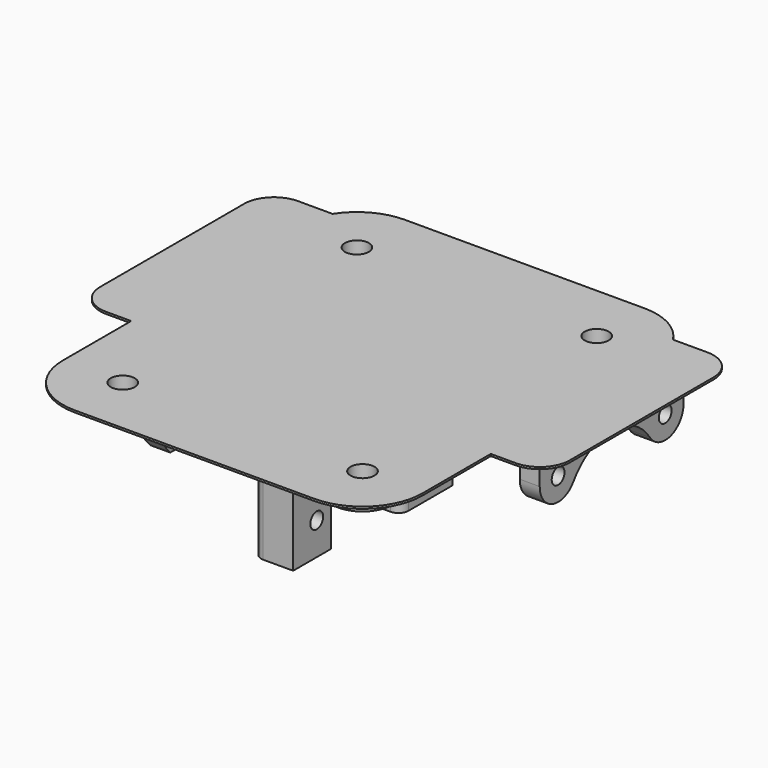
from build123d import *

# Parameters (mm, degrees)
F1_R          = 1.2
F2_DEPTH      = 2
F3_R          = 2
F4_W          = 4
F4_H          = 4.75
F5_DEPTH      = 9
F6_W          = 8.8
F6_H          = 2
F6_W_2        = 2
F6_H_2        = 6.5
F7_DEPTH      = 4
F8_R          = 0.8
F9_DEPTH      = 4
F10_T4_DEPTH  = 2
F10_S5_R      = 0.8
F10_T6_DEPTH  = 3
F10_T10_DEPTH = 6.5
F10_T15_DEPTH = 6.5
F10_T20_DEPTH = 2
F10_S21_R     = 0.8
F10_T22_DEPTH = 3
F10_T27_DEPTH = 6.5
F10_S29_R     = 0.8
F10_T30_DEPTH = 5
F10_T33_DEPTH = 4.5
F10_T40_DEPTH = 4.5
F10_T44_DEPTH = 6.5
F10_S46_R     = 0.8
F10_T47_DEPTH = 5
F10_T49_DEPTH = 6.5
F10_T51_DEPTH = 11.5
F11_W         = 2
F11_H         = 18
F12_DEPTH     = 12
F13_R         = 1.55
F13_R_2       = 0.8
F14_DEPTH     = 2
F15_R         = 0.8
F16_DEPTH     = 2
F19_DEPTH     = 0.2
F20_W         = 20.8
F20_H         = 21.9
F21_DEPTH     = 0.4


# Not quite as in the source:
# - a fillet or chamfer that OpenCascade refuses, or shapes differently, is made with other operations: its cross-section is extruded or revolved along the edge and cut away or added
# - two fillets or chamfers of one size are made in one step


with BuildPart() as f2:
    # F1 (on Top) → F2 (new body)
    with BuildSketch(Plane.XY):
        with BuildLine():
            Line((-4.2895651858, 24.55), (-9.8, 24.55))
            Line((-9.8, 24.55), (-9.8, 6.55))
            Line((-9.8, 6.55), (-4.3, 6.55))
            Line((-4.3, 6.55), (-4.3, -5))
            ThreePointArc((-4.3, -5), (-3.4213203436, -7.1213203436), (-1.3, -8))
            Line((-1.3, -8), (22.7, -8))
            ThreePointArc((22.7, -8), (24.8213203436, -7.1213203436), (25.7, -5))
            Line((25.7, -5), (25.7, 6.55))
            Line((25.7, 6.55), (31.2, 6.55))
            Line((31.2, 6.55), (31.2, 24.55))
            Line((31.2, 24.55), (25.6895651858, 24.55))
            ThreePointArc((25.6895651858, 24.55), (24.7310096012, 26.5079402166), (22.7, 27.3))
            Line((22.7, 27.3), (-1.3, 27.3))
            ThreePointArc((-1.3, 27.3), (-3.3310096012, 26.5079402166), (-4.2895651858, 24.55))
        make_face()
        with Locations((-1.3, -5)):
            Circle(F1_R, mode=Mode.SUBTRACT)
        with Locations((22.7, -5)):
            Circle(F1_R, mode=Mode.SUBTRACT)
        with Locations((-1.3, 24.3)):
            Circle(F1_R, mode=Mode.SUBTRACT)
        with Locations((22.7, 24.3)):
            Circle(F1_R, mode=Mode.SUBTRACT)
    extrude(amount=F2_DEPTH)

    # F3
    f3_edges = [f2.edges().sort_by_distance(p)[0] for p in [
        (-4.289565, 24.55, 1),
        (-4.3, 6.55, 1),
        (25.7, 6.55, 1),
        (25.689565, 24.55, 1),
    ]]
    fillet(f3_edges, radius=F3_R)

    # F4 (on face) → F5 (join)
    with BuildSketch(Plane(origin=(0, 0, 0), x_dir=(1, 0, 0), z_dir=(0, 0, -1))):
        with Locations((13.8, 2.675)):
            Rectangle(F4_W, F4_H)
        with Locations((13.8, -23.975)):
            Rectangle(F4_W, F4_H)
    extrude(amount=F5_DEPTH)

    # F6 (on face) → F7 (join)
    with BuildSketch(Plane(origin=(0, 0, 0), x_dir=(1, 0, 0), z_dir=(0, 0, -1))):
        Polygon((-2.3, -18.3), (-0.3, -18.3), (-0.3, 0.3), (11.8, 0.3), (11.8, 2.3), (-2.3, 2.3), align=None)
        with Locations((7.4, -22.6)):
            Rectangle(F6_W, F6_H)
        with Locations((21.5, -3.25)):
            Rectangle(F6_W_2, F6_H_2)
    extrude(amount=F7_DEPTH)

    # F8 (on face) → F9 (cut, through all)
    with BuildSketch(Plane.YZ.offset(15.8)):
        with Locations((23.4, -5.75)):
            Circle(F8_R)
        with Locations((-2.1, -5.75)):
            Circle(F8_R)
    extrude(amount=-F9_DEPTH, mode=Mode.SUBTRACT)

    # F10: fillet of radius 1 on 10 edges, made by hand


with BuildPart() as f10_tool2:
    # F10_s3 → F10_t4 (new body)
    with BuildSketch(Plane.XZ.offset(0.3)):
        with BuildLine():
            ThreePointArc((11.8, -5), (11.5071067812, -4.2928932188), (10.8, -4))
            Line((10.8, -4), (11.8, -4))
            Line((11.8, -4), (11.8, -5))
        make_face()
    extrude(amount=F10_T4_DEPTH)

    # F10_s5 → F10_t6 (cut, symmetric)
    with BuildSketch(Plane.YZ.offset(11.3)):
        with Locations((-2.1, -5.75)):
            Circle(F10_S5_R)
    extrude(amount=F10_T6_DEPTH, both=True, mode=Mode.SUBTRACT)


with BuildPart() as f2_1:
    add(f2.part)

    # F10_t1: union F10_tool2
    add(f10_tool2.part)


with BuildPart() as f10_tool8:
    # F10_s9 → F10_t10 (new body)
    with BuildSketch(Plane.XY.offset(2.5)):
        with BuildLine():
            ThreePointArc((11.8, -3.3), (11.5071067812, -2.5928932188), (10.8, -2.3))
            Line((10.8, -2.3), (11.8, -2.3))
            Line((11.8, -2.3), (11.8, -3.3))
        make_face()
    extrude(amount=-F10_T10_DEPTH)

    split(bisect_by=Plane.XY.offset(2), keep=Keep.BOTTOM)


with BuildPart() as f2_2:
    add(f2_1.part)

    # F10_t7: union F10_tool8
    add(f10_tool8.part)


with BuildPart() as f10_tool13:
    # F10_s14 → F10_t15 (new body)
    with BuildSketch(Plane.XY.offset(2.5)):
        with BuildLine():
            ThreePointArc((11.8, 24.6), (11.5071067812, 23.8928932188), (10.8, 23.6))
            Line((10.8, 23.6), (11.8, 23.6))
            Line((11.8, 23.6), (11.8, 24.6))
        make_face()
    extrude(amount=-F10_T15_DEPTH)

    split(bisect_by=Plane.XY.offset(2), keep=Keep.BOTTOM)


with BuildPart() as f2_3:
    add(f2_2.part)

    # F10_t12: union F10_tool13
    add(f10_tool13.part)


with BuildPart() as f10_tool18:
    # F10_s19 → F10_t20 (new body)
    with BuildSketch(Plane.XZ.offset(-23.6)):
        with BuildLine():
            ThreePointArc((11.8, -5), (11.5071067812, -4.2928932188), (10.8, -4))
            Line((10.8, -4), (11.8, -4))
            Line((11.8, -4), (11.8, -5))
        make_face()
    extrude(amount=F10_T20_DEPTH)

    # F10_s21 → F10_t22 (cut, symmetric)
    with BuildSketch(Plane.YZ.offset(11.3)):
        with Locations((23.4, -5.75)):
            Circle(F10_S21_R)
    extrude(amount=F10_T22_DEPTH, both=True, mode=Mode.SUBTRACT)


with BuildPart() as f2_4:
    add(f2_3.part)

    # F10_t17: union F10_tool18
    add(f10_tool18.part)


with BuildPart() as f10_tool25:
    # F10_s26 → F10_t27 (new body)
    with BuildSketch(Plane.XY):
        with BuildLine():
            ThreePointArc((11.8, -3.3), (11.5071067812, -2.5928932188), (10.8, -2.3))
            Line((10.8, -2.3), (11.8, -2.3))
            Line((11.8, -2.3), (11.8, -3.3))
        make_face()
    extrude(amount=-F10_T27_DEPTH)

    split(bisect_by=Plane.XY.offset(-4), keep=Keep.BOTTOM)

    # F10_s29 → F10_t30 (cut, symmetric)
    with BuildSketch(Plane.YZ.offset(11.3)):
        with Locations((-2.1, -5.75)):
            Circle(F10_S29_R)
    extrude(amount=F10_T30_DEPTH, both=True, mode=Mode.SUBTRACT)


with BuildPart() as f10_tool31:
    # F10_s32 → F10_t33 (new body)
    with BuildSketch(Plane.XZ.offset(0.3)):
        with BuildLine():
            ThreePointArc((11.8, -5), (11.5071067812, -4.2928932188), (10.8, -4))
            Line((10.8, -4), (11.8, -4))
            Line((11.8, -4), (11.8, -5))
        make_face()
    extrude(amount=F10_T33_DEPTH)

    split(bisect_by=Plane.XZ.offset(2.3), keep=Keep.TOP)


with BuildPart() as f10_tool25_1:
    add(f10_tool25.part)

    # F10_t35: intersect F10_tool31
    add(f10_tool31.part, mode=Mode.INTERSECT)


with BuildPart() as f2_5:
    add(f2_4.part)

    # F10_t23: union F10_tool25
    add(f10_tool25_1.part)


with BuildPart() as f10_tool38:
    # F10_s39 → F10_t40 (new body)
    with BuildSketch(Plane.XZ.offset(-26.1)):
        with BuildLine():
            ThreePointArc((11.8, -5), (11.5071067812, -4.2928932188), (10.8, -4))
            Line((10.8, -4), (11.8, -4))
            Line((11.8, -4), (11.8, -5))
        make_face()
    extrude(amount=F10_T40_DEPTH)

    split(bisect_by=Plane.XZ.offset(-23.6), keep=Keep.BOTTOM)


with BuildPart() as f10_tool42:
    # F10_s43 → F10_t44 (new body)
    with BuildSketch(Plane.XY):
        with BuildLine():
            ThreePointArc((11.8, 24.6), (11.5071067812, 23.8928932188), (10.8, 23.6))
            Line((10.8, 23.6), (11.8, 23.6))
            Line((11.8, 23.6), (11.8, 24.6))
        make_face()
    extrude(amount=-F10_T44_DEPTH)

    split(bisect_by=Plane.XY.offset(-4), keep=Keep.BOTTOM)

    # F10_s46 → F10_t47 (cut, symmetric)
    with BuildSketch(Plane.YZ.offset(11.3)):
        with Locations((23.4, -5.75)):
            Circle(F10_S46_R)
    extrude(amount=F10_T47_DEPTH, both=True, mode=Mode.SUBTRACT)


with BuildPart() as f10_tool38_1:
    add(f10_tool38.part)

    # F10_t48: intersect F10_tool42
    add(f10_tool42.part, mode=Mode.INTERSECT)


with BuildPart() as f2_6:
    add(f2_5.part)

    # F10_t36: union F10_tool38
    add(f10_tool38_1.part)

    # F10_s50 → F10_t49 (cut)
    with BuildSketch(Plane.XY.offset(-6.5)):
        with BuildLine():
            ThreePointArc((-1.3, -2.3), (-2.0071067812, -2.0071067812), (-2.3, -1.3))
            Line((-2.3, -1.3), (-2.3, -2.3))
            Line((-2.3, -2.3), (-1.3, -2.3))
        make_face()
        with BuildLine():
            ThreePointArc((-2.3, 17.3), (-2.0071067812, 18.0071067812), (-1.3, 18.3))
            Line((-1.3, 18.3), (-2.3, 18.3))
            Line((-2.3, 18.3), (-2.3, 17.3))
        make_face()
        with BuildLine():
            ThreePointArc((3, 22.6), (3.2928932188, 23.3071067812), (4, 23.6))
            Line((4, 23.6), (3, 23.6))
            Line((3, 23.6), (3, 22.6))
        make_face()
        with BuildLine():
            ThreePointArc((21.5, 0), (22.2071067812, 0.2928932188), (22.5, 1))
            Line((22.5, 1), (22.5, 0))
            Line((22.5, 0), (21.5, 0))
        make_face()
    extrude(amount=F10_T49_DEPTH, mode=Mode.SUBTRACT)

    # F10_s52 → F10_t51 (cut)
    with BuildSketch(Plane.XY.offset(-11.5)):
        with BuildLine():
            ThreePointArc((11.8, 25.35), (12.0928932188, 26.0571067812), (12.8, 26.35))
            Line((12.8, 26.35), (11.8, 26.35))
            Line((11.8, 26.35), (11.8, 25.35))
        make_face()
        with BuildLine():
            ThreePointArc((12.8, -5.05), (12.0928932188, -4.7571067812), (11.8, -4.05))
            Line((11.8, -4.05), (11.8, -5.05))
            Line((11.8, -5.05), (12.8, -5.05))
        make_face()
    extrude(amount=F10_T51_DEPTH, mode=Mode.SUBTRACT)

    # F11 (on face) → F12 (join)
    with BuildSketch(Plane(origin=(0, 0, 0), x_dir=(1, 0, 0), z_dir=(0, 0, -1))):
        with Locations((-8.8, -15.55)):
            Rectangle(F11_W, F11_H)
        with Locations((30.2, -15.55)):
            Rectangle(F11_W, F11_H)
    extrude(amount=F12_DEPTH)

    # F13 (on face) → F14 (cut, through all)
    with BuildSketch(Plane(origin=(-9.8, 0, 0), x_dir=(0, -1, 0), z_dir=(-1, 0, 0))):
        with Locations((-15.55, -5.75)):
            Circle(F13_R)
        with Locations((-21.55, -5.75)):
            Circle(F13_R_2)
        with Locations((-9.55, -5.75)):
            Circle(F13_R_2)
        with BuildLine():
            ThreePointArc((-22.0259169235, -12), (-23.8951558497, -9.1202186642), (-24.55, -5.75))
            Line((-24.55, -5.75), (-24.55, -12))
            Line((-24.55, -12), (-22.0259169235, -12))
        make_face()
        with BuildLine():
            ThreePointArc((-6.55, -5.75), (-7.2048441503, -9.1202186642), (-9.0740830765, -12))
            Line((-9.0740830765, -12), (-6.55, -12))
            Line((-6.55, -12), (-6.55, -5.75))
        make_face()
    extrude(amount=-F14_DEPTH, mode=Mode.SUBTRACT)

    # F15 (on face) → F16 (cut, through all)
    with BuildSketch(Plane.YZ.offset(31.2)):
        with BuildLine():
            ThreePointArc((24.55, -1.2876575658), (22.9160115829, -3.4891181199), (20.3357142857, -2.562612547))
            ThreePointArc((20.3357142857, -2.562612547), (15.55, 0), (10.7642857143, -2.562612547))
            ThreePointArc((10.7642857143, -2.562612547), (8.1839884171, -3.4891181199), (6.55, -1.2876575658))
            Line((6.55, -1.2876575658), (6.55, -12))
            Line((6.55, -12), (24.55, -12))
            Line((24.55, -12), (24.55, -1.2876575658))
        make_face()
        with Locations((8.85, -1.2876575658)):
            Circle(F15_R)
        with Locations((22.25, -1.2876575658)):
            Circle(F15_R)
    extrude(amount=-F16_DEPTH, mode=Mode.SUBTRACT)

    # F18 (on face) → F19 (join)
    with BuildSketch(Plane.XY.offset(2)):
        with BuildLine():
            ThreePointArc((-9.8, 27.55), (-11.9213203436, 26.6713203436), (-12.8, 24.55))
            Line((-12.8, 24.55), (-12.8, 6.55))
            ThreePointArc((-12.8, 6.55), (-11.9213203436, 4.4286796564), (-9.8, 3.55))
            Line((-9.8, 3.55), (-7.3, 3.55))
            Line((-7.3, 3.55), (-7.3, -5))
            ThreePointArc((-7.3, -5), (-5.5426406871, -9.2426406871), (-1.3, -11))
            Line((-1.3, -11), (22.7, -11))
            ThreePointArc((22.7, -11), (26.9426406871, -9.2426406871), (28.7, -5))
            Line((28.7, -5), (28.7, 3.55))
            Line((28.7, 3.55), (31.2, 3.55))
            ThreePointArc((31.2, 3.55), (33.3213203436, 4.4286796564), (34.2, 6.55))
            Line((34.2, 6.55), (34.2, 24.55))
            ThreePointArc((34.2, 24.55), (33.3213203436, 26.6713203436), (31.2, 27.55))
            Line((31.2, 27.55), (27.7435602505, 27.55))
            ThreePointArc((27.7435602505, 27.55), (25.5722813233, 29.5678268764), (22.7, 30.3))
            Line((22.7, 30.3), (-1.3, 30.3))
            ThreePointArc((-1.3, 30.3), (-4.1722813233, 29.5678268764), (-6.3435602505, 27.55))
            Line((-6.3435602505, 27.55), (-9.8, 27.55))
        make_face()
        with BuildLine():
            Line((-9.8, 6.55), (-9.8, 24.55))
            Line((-9.8, 24.55), (-5.7651427749, 24.55))
            ThreePointArc((-5.7651427749, 24.55), (-4.7163339267, 24.8470613634), (-3.9790856649, 25.65))
            ThreePointArc((-3.9790856649, 25.65), (-2.8732132723, 26.8544079549), (-1.3, 27.3))
            Line((-1.3, 27.3), (22.7, 27.3))
            ThreePointArc((22.7, 27.3), (24.2732132723, 26.8544079549), (25.3790856649, 25.65))
            ThreePointArc((25.3790856649, 25.65), (26.1163339267, 24.8470613634), (27.1651427749, 24.55))
            Line((27.1651427749, 24.55), (31.2, 24.55))
            Line((31.2, 24.55), (31.2, 6.55))
            Line((31.2, 6.55), (27.7, 6.55))
            ThreePointArc((27.7, 6.55), (26.2857864376, 5.9642135624), (25.7, 4.55))
            Line((25.7, 4.55), (25.7, -5))
            ThreePointArc((25.7, -5), (24.8213203436, -7.1213203436), (22.7, -8))
            Line((22.7, -8), (-1.3, -8))
            ThreePointArc((-1.3, -8), (-3.4213203436, -7.1213203436), (-4.3, -5))
            Line((-4.3, -5), (-4.3, 4.55))
            ThreePointArc((-4.3, 4.55), (-4.8857864376, 5.9642135624), (-6.3, 6.55))
            Line((-6.3, 6.55), (-9.8, 6.55))
        make_face(mode=Mode.SUBTRACT)
    extrude(amount=-F19_DEPTH)

    # F20 (on face) → F21 (cut)
    with BuildSketch(Plane(origin=(0, 0, 0), x_dir=(1, 0, 0), z_dir=(0, 0, -1))):
        with Locations((10.1, -10.65)):
            Rectangle(F20_W, F20_H)
    extrude(amount=-F21_DEPTH, mode=Mode.SUBTRACT)


solid = f2_6.part
